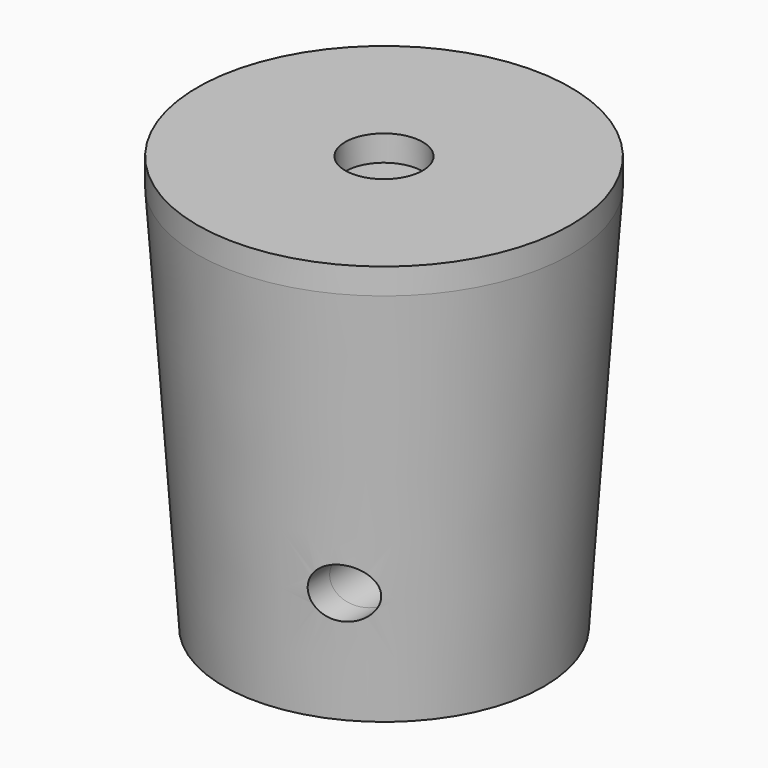
from build123d import *

# Parameters (mm, degrees)
F5_D       = 50.8
F5_DEPTH   = 183.761479
F5_2_D     = 50.8
F5_2_DEPTH = 183.761479
F7_D       = 76.2


with BuildPart() as f1:
    # F0 (on Front) → F1 (revolve)
    with BuildSketch(Plane.XZ):
        Polygon((0, -118.385883), (0, -156.485883), (133.764577, -156.485883), (158.121877, 198.176414), (158.300649, 200.779488), (120.110904, 200.779488), (101.538188, -69.654506), (98.191442, -118.385883), (50.8, -118.385883), align=None)
    revolve(axis=Axis((0, 0, 67.959784), (0, 0, 1)))

    # F5 (through all, one way)
    with BuildSketch(Plane(origin=(0, 0, 0), x_dir=(1, 0, 0), z_dir=(0, 1, 0))):
        with Locations((76.197878, 67.914199)):
            Circle(F5_D / 2)
    extrude(amount=-F5_DEPTH, mode=Mode.SUBTRACT)


with BuildPart() as f2:
    # F0 (on Front) → F2 (revolve)
    with BuildSketch(Plane.XZ):
        Polygon((0, -156.485883), (0, -181.885883), (157.48, -181.885883), (183.760479, 200.779488), (158.300649, 200.779488), (158.121877, 198.176414), (133.764577, -156.485883), align=None)
    revolve(axis=Axis((0, 0, 67.959784), (0, 0, 1)))

    # F5#2 (through all, one way)
    with BuildSketch(Plane(origin=(0, 0, 0), x_dir=(1, 0, 0), z_dir=(0, 1, 0))):
        with Locations((76.197878, 67.914199)):
            Circle(F5_2_D / 2)
    extrude(amount=-F5_2_DEPTH, mode=Mode.SUBTRACT)


with BuildPart() as f3:
    # F0 (on Front) → F3 (revolve)
    with BuildSketch(Plane.XZ):
        with BuildLine():
            Line((0, -67.585883), (0, -118.385883))
            Line((0, -118.385883), (50.8, -118.385883))
            Line((50.8, -118.385883), (50.8, -68.242514))
            ThreePointArc((50.8, -68.242514), (50.797878, -67.914199), (50.8, -67.585883))
            Line((50.8, -67.585883), (0, -67.585883))
        make_face()
    revolve(axis=Axis((0, 0, 67.959784), (0, 0, 1)))


with BuildPart() as f4:
    # F0 (on Front) → F4 (revolve)
    with BuildSketch(Plane.XZ):
        Polygon((158.300649, 200.779488), (183.760479, 200.779488), (183.584616, 226.179488), (0, 226.179488), (0, 200.779488), (120.110904, 200.779488), align=None)
    revolve(axis=Axis((0, 0, 67.959784), (0, 0, 1)))

    # F7 (through all)
    with Locations(Plane.XY.offset(226.179488)):
        with Locations((0, 0)):
            Hole(F7_D / 2)


with BuildPart() as f9:
    # F8 (on Front) → F9 (revolve)
    with BuildSketch(Plane.XZ):
        with BuildLine():
            Line((0, -54.885883), (0, -67.585883))
            Line((0, -67.585883), (38.1, -67.585883))
            ThreePointArc((38.1, -67.585883), (51.197012, -62.381575), (57.15, -49.607441))
            Line((57.15, -49.607441), (66.04, 103.864117))
            Line((66.04, 103.864117), (53.318711, 103.864117))
            Line((53.318711, 103.864117), (45.225828, -35.846494))
            ThreePointArc((45.225828, -35.846494), (38.921541, -49.374457), (25.051646, -54.885883))
            Line((25.051646, -54.885883), (0, -54.885883))
        make_face()
    revolve(axis=Axis((0, 0, -61.235883), (0, 0, -1)))


solid = Compound([f1.part, f2.part, f3.part, f4.part, f9.part])
